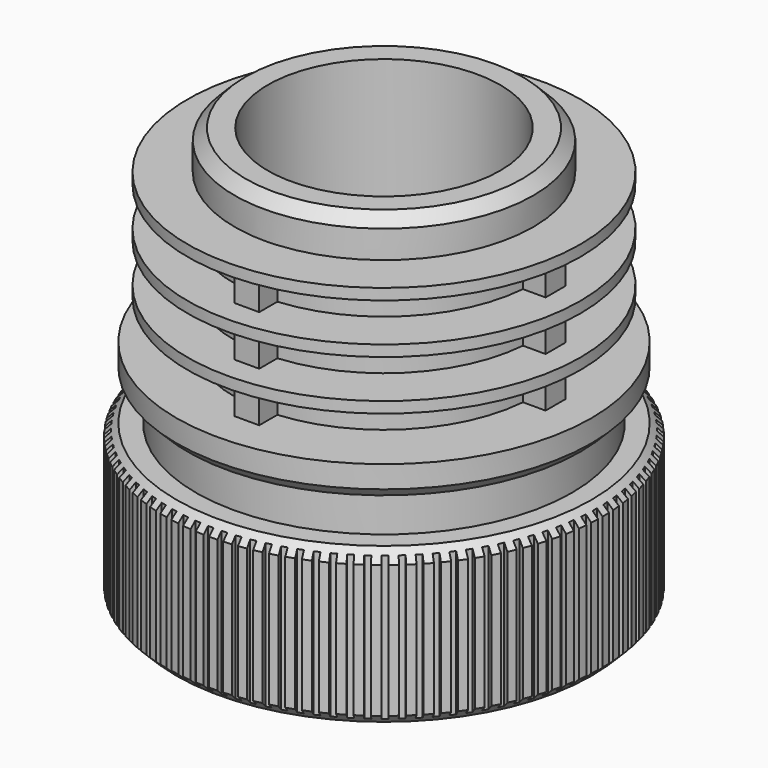
from build123d import *

# Parameters (mm, degrees)
F3_SIZE  = 1
F4_START = -3.5
F4_DEPTH = 21.5
F5_DEPTH = 37.501
F2_R     = 10.5
F6_DEPTH = 33


# Not quite as in the source:
# - a feature names something its author has since deleted; it is built from what else it names


with BuildPart() as f1:
    # F0 (on Front) → F1 (revolve)
    with BuildSketch(Plane.XZ):
        Polygon((0, 0), (19.75, 0), (19.75, 14), (17, 14), (17, 17.5), (18.75, 17.5), (18.75, 20.5), (13.5, 20.5), (13.5, 24), (17.75, 24), (17.75, 25), (13.5, 25), (13.5, 28.5), (17.75, 28.5), (17.75, 29.5), (13.5, 29.5), (13.5, 33), (17.75, 33), (17.75, 34), (13.5, 34), (13.5, 37.5), (0, 37.5), align=None)
    revolve(axis=Axis((0, 0, 18.75), (0, 0, -1)))

    # F3
    f3_edges = [f1.edges().sort_by_distance(p)[0] for p in [
        (-19.75, 0, 14),
        (-18.75, 0, 17.5),
        (-19.75, 0, 0),
        (-13.5, 0, 37.5),
    ]]
    chamfer(f3_edges, length=F3_SIZE)

    # F2 (on face) → F4 (join)
    with BuildSketch(Plane.XY.offset(37.5).offset(F4_START)):
        with BuildLine():
            Line((1.125, -15.5), (1.125, -13.453043336))
            ThreePointArc((1.125, -13.453043336), (0, -13.5), (-1.125, -13.453043336))
            Line((-1.125, -13.453043336), (-1.125, -15.5))
            Line((-1.125, -15.5), (1.125, -15.5))
        make_face()
        with BuildLine():
            ThreePointArc((-13.453043336, -1.125), (-13.5, 0), (-13.453043336, 1.125))
            Line((-13.453043336, 1.125), (-15.5, 1.125))
            Line((-15.5, 1.125), (-15.5, -1.125))
            Line((-15.5, -1.125), (-13.453043336, -1.125))
        make_face()
        with BuildLine():
            ThreePointArc((-1.125, 13.453043336), (0, 13.5), (1.125, 13.453043336))
            Line((1.125, 13.453043336), (1.125, 15.5))
            Line((1.125, 15.5), (-1.125, 15.5))
            Line((-1.125, 15.5), (-1.125, 13.453043336))
        make_face()
        with BuildLine():
            ThreePointArc((13.453043336, 1.125), (13.4882557256, 0.5629897708), (13.5, 0))
            ThreePointArc((13.5, 0), (13.4882557256, -0.5629897708), (13.453043336, -1.125))
            Line((13.453043336, -1.125), (15.5, -1.125))
            Line((15.5, -1.125), (15.5, 1.125))
            Line((15.5, 1.125), (13.453043336, 1.125))
        make_face()
    extrude(amount=-F4_DEPTH)

    # F2 (on face) → F5 (cut, through all)
    with BuildSketch(Plane.XY.offset(37.5)):
        with BuildLine():
            Line((-3.1159466804, 19.0027202338), (-3.2084511899, 19.4876458548))
            ThreePointArc((-3.2084511899, 19.4876458548), (-3.454892922, 19.4454677212), (-3.7007809631, 19.4001732019))
            Line((-3.7007809631, 19.4001732019), (-3.6070903058, 18.9090295765))
            Line((-3.6070903058, 18.9090295765), (-3.1159466804, 19.0027202338))
        make_face()
        with BuildLine():
            ThreePointArc((-16.2668570836, -11.2005294795), (-16.1237633813, -11.4055580497), (-15.9780856389, -11.6087587328))
            Line((-15.9780856389, -11.6087587328), (-15.5735771417, -11.3148661066))
            Line((-15.5735771417, -11.3148661066), (-15.8674697679, -10.9103576094))
            Line((-15.8674697679, -10.9103576094), (-16.2668570836, -11.2005294795))
        make_face()
        with BuildLine():
            ThreePointArc((-13.8799563847, -14.0502423736), (-13.7009787423, -14.2248262381), (-13.5198053421, -14.3971303916))
            Line((-13.5198053421, -14.3971303916), (-13.1775317891, -14.0326460779))
            Line((-13.1775317891, -14.0326460779), (-13.5420161028, -13.6903725249))
            Line((-13.5420161028, -13.6903725249), (-13.8799563847, -14.0502423736))
        make_face()
        with BuildLine():
            ThreePointArc((-12.9703454432, -14.8940471022), (-12.7807587607, -15.0570483661), (-12.5891237975, -15.2176365448))
            Line((-12.5891237975, -15.2176365448), (-12.2704118027, -14.8323799234))
            Line((-12.2704118027, -14.8323799234), (-12.6556684241, -14.5136679286))
            Line((-12.6556684241, -14.5136679286), (-12.9703454432, -14.8940471022))
        make_face()
        with BuildLine():
            ThreePointArc((15.6790718313, -12.0095464739), (15.8298472032, -11.8100989633), (15.9780856389, -11.6087587328))
            Line((15.9780856389, -11.6087587328), (15.5735771417, -11.3148661066))
            Line((15.5735771417, -11.3148661066), (15.2796845156, -11.7193746038))
            Line((15.2796845156, -11.7193746038), (15.6790718313, -12.0095464739))
        make_face()
        with BuildLine():
            ThreePointArc((17.651716969, -8.8588592971), (17.7624489578, -8.6346920629), (17.8703342862, -8.4091410084))
            Line((17.8703342862, -8.4091410084), (17.41792076, -8.1962513626))
            Line((17.41792076, -8.1962513626), (17.2050311142, -8.6486648889))
            Line((17.2050311142, -8.6486648889), (17.651716969, -8.8588592971))
        make_face()
        with BuildLine():
            ThreePointArc((18.1731377154, -7.7330178828), (18.2695756229, -7.5023400723), (18.3630855963, -7.2704599155))
            Line((18.3630855963, -7.2704599155), (17.8981973533, -7.0863976392))
            Line((17.8981973533, -7.0863976392), (17.714135077, -7.5512858821))
            Line((17.714135077, -7.5512858821), (18.1731377154, -7.7330178828))
        make_face()
        with BuildLine():
            Line((0.5, 19.25), (0.5, 19.7436698716))
            ThreePointArc((0.5, 19.7436698716), (0.2500200345, 19.7484174045), (0, 19.75))
            Line((0, 19.75), (0, 19.25))
            Line((0, 19.25), (0.5, 19.25))
        make_face()
        with BuildLine():
            Line((9.7119115665, 16.6280267538), (9.9497388409, 17.06063296))
            ThreePointArc((9.9497388409, 17.06063296), (9.7329668687, 17.1852220217), (9.5146350635, 17.3070569309))
            Line((9.5146350635, 17.3070569309), (9.2737582265, 16.8689035908))
            Line((9.2737582265, 16.8689035908), (9.7119115665, 16.6280267538))
        make_face()
        with BuildLine():
            Line((8.6486648889, 17.2050311142), (8.8588592971, 17.651716969))
            ThreePointArc((8.8588592971, 17.651716969), (8.6346920629, 17.7624489578), (8.4091410084, 17.8703342862))
            Line((8.4091410084, 17.8703342862), (8.1962513626, 17.41792076))
            Line((8.1962513626, 17.41792076), (8.6486648889, 17.2050311142))
        make_face()
        with BuildLine():
            Line((6.4241053999, 18.1533294415), (6.5766577798, 18.6228373898))
            ThreePointArc((6.5766577798, 18.6228373898), (6.340379773, 18.7046006195), (6.1030856389, 18.7833661968))
            Line((6.1030856389, 18.7833661968), (5.9485771417, 18.3078379387))
            Line((5.9485771417, 18.3078379387), (6.4241053999, 18.1533294415))
        make_face()
        with BuildLine():
            Line((5.2715719085, 18.5208809081), (5.3943426132, 18.999041233))
            ThreePointArc((5.3943426132, 18.999041233), (5.1533968913, 19.0658071028), (4.9116252715, 19.1295174323))
            Line((4.9116252715, 19.1295174323), (4.7872803279, 18.6452258517))
            Line((4.7872803279, 18.6452258517), (5.2715719085, 18.5208809081))
        make_face()
        with BuildLine():
            Line((-1.9166073955, 19.1608746171), (-1.9784806368, 19.6506517543))
            ThreePointArc((-1.9784806368, 19.6506517543), (-2.2270844593, 19.6240310541), (-2.4753313629, 19.594265351))
            Line((-2.4753313629, 19.594265351), (-2.4126647461, 19.0982080003))
            Line((-2.4126647461, 19.0982080003), (-1.9166073955, 19.1608746171))
        make_face()
        with BuildLine():
            Line((-4.3029887474, 18.7695707953), (-4.425759452, 19.2477311201))
            ThreePointArc((-4.425759452, 19.2477311201), (-4.6690665007, 19.1901620111), (-4.9116252715, 19.1295174323))
            Line((-4.9116252715, 19.1295174323), (-4.7872803279, 18.6452258517))
            Line((-4.7872803279, 18.6452258517), (-4.3029887474, 18.7695707953))
        make_face()
        with BuildLine():
            ThreePointArc((-15.531471092, -12.1998322005), (-15.3757859019, -12.3954712657), (-15.2176365448, -12.5891237975))
            Line((-15.2176365448, -12.5891237975), (-14.8323799234, -12.2704118027))
            Line((-14.8323799234, -12.2704118027), (-15.1510919183, -11.8851551813))
            Line((-15.1510919183, -11.8851551813), (-15.531471092, -12.1998322005))
        make_face()
        with BuildLine():
            ThreePointArc((-14.7347894795, -13.1509877573), (-14.5671272201, -13.3364652196), (-14.3971303916, -13.5198053421))
            Line((-14.3971303916, -13.5198053421), (-14.0326460779, -13.1775317891))
            Line((-14.0326460779, -13.1775317891), (-14.3749196308, -12.8130474754))
            Line((-14.3749196308, -12.8130474754), (-14.7347894795, -13.1509877573))
        make_face()
        with BuildLine():
            ThreePointArc((12.1998322005, -15.531471092), (12.3954712657, -15.3757859019), (12.5891237975, -15.2176365448))
            Line((12.5891237975, -15.2176365448), (12.2704118027, -14.8323799234))
            Line((12.2704118027, -14.8323799234), (11.8851551813, -15.1510919183))
            Line((11.8851551813, -15.1510919183), (12.1998322005, -15.531471092))
        make_face()
        with BuildLine():
            ThreePointArc((13.1509877573, -14.7347894795), (13.3364652196, -14.5671272201), (13.5198053421, -14.3971303916))
            Line((13.5198053421, -14.3971303916), (13.1775317891, -14.0326460779))
            Line((13.1775317891, -14.0326460779), (12.8130474754, -14.3749196308))
            Line((12.8130474754, -14.3749196308), (13.1509877573, -14.7347894795))
        make_face()
        with BuildLine():
            Line((18.7695707953, 4.3029887474), (19.2477311201, 4.425759452))
            ThreePointArc((19.2477311201, 4.425759452), (19.1901620111, 4.6690665007), (19.1295174323, 4.9116252715))
            Line((19.1295174323, 4.9116252715), (18.6452258517, 4.7872803279))
            Line((18.6452258517, 4.7872803279), (18.7695707953, 4.3029887474))
        make_face()
        with BuildLine():
            ThreePointArc((14.0502423736, -13.8799563847), (14.2248262381, -13.7009787423), (14.3971303916, -13.5198053421))
            Line((14.3971303916, -13.5198053421), (14.0326460779, -13.1775317891))
            Line((14.0326460779, -13.1775317891), (13.6903725249, -13.5420161028))
            Line((13.6903725249, -13.5420161028), (14.0502423736, -13.8799563847))
        make_face()
        with BuildLine():
            ThreePointArc((14.8940471022, -12.9703454432), (15.0570483661, -12.7807587607), (15.2176365448, -12.5891237975))
            Line((15.2176365448, -12.5891237975), (14.8323799234, -12.2704118027))
            Line((14.8323799234, -12.2704118027), (14.5136679286, -12.6556684241))
            Line((14.5136679286, -12.6556684241), (14.8940471022, -12.9703454432))
        make_face()
        with BuildLine():
            Line((-19.25, 0.5), (-19.7436698716, 0.5))
            ThreePointArc((-19.7436698716, 0.5), (-19.7484174045, 0.2500200345), (-19.75, 0))
            Line((-19.75, 0), (-19.25, 0))
            Line((-19.25, 0), (-19.25, 0.5))
        make_face()
        with BuildLine():
            Line((-12.8130474754, 14.3749196308), (-13.1509877573, 14.7347894795))
            ThreePointArc((-13.1509877573, 14.7347894795), (-13.3364652196, 14.5671272201), (-13.5198053421, 14.3971303916))
            Line((-13.5198053421, 14.3971303916), (-13.1775317891, 14.0326460779))
            Line((-13.1775317891, 14.0326460779), (-12.8130474754, 14.3749196308))
        make_face()
        with BuildLine():
            ThreePointArc((-6.5766577798, -18.6228373898), (-6.340379773, -18.7046006195), (-6.1030856389, -18.7833661968))
            Line((-6.1030856389, -18.7833661968), (-5.9485771417, -18.3078379387))
            Line((-5.9485771417, -18.3078379387), (-6.4241053999, -18.1533294415))
            Line((-6.4241053999, -18.1533294415), (-6.5766577798, -18.6228373898))
        make_face()
        with BuildLine():
            Line((-0.7097041367, 19.243409782), (-0.7407019244, 19.7361055089))
            ThreePointArc((-0.7407019244, 19.7361055089), (-0.9904867117, 19.7251473017), (-1.2401127607, 19.7110278865))
            Line((-1.2401127607, 19.7110278865), (-1.2087175009, 19.2120145222))
            Line((-1.2087175009, 19.2120145222), (-0.7097041367, 19.243409782))
        make_face()
        with BuildLine():
            Line((7.5512858821, 17.714135077), (7.7330178828, 18.1731377154))
            ThreePointArc((7.7330178828, 18.1731377154), (7.5023400723, 18.2695756229), (7.2704599155, 18.3630855963))
            Line((7.2704599155, 18.3630855963), (7.0863976392, 17.8981973533))
            Line((7.0863976392, 17.8981973533), (7.5512858821, 17.714135077))
        make_face()
        with BuildLine():
            ThreePointArc((-1.7387286529, -19.6733149894), (-1.4895400657, -19.693749526), (-1.2401127607, -19.7110278865))
            Line((-1.2401127607, -19.7110278865), (-1.2087175009, -19.2120145222))
            Line((-1.2087175009, -19.2120145222), (-1.7077308652, -19.1806192625))
            Line((-1.7077308652, -19.1806192625), (-1.7387286529, -19.6733149894))
        make_face()
        with BuildLine():
            ThreePointArc((-4.1907384407, -19.3002645402), (-3.9460759065, -19.3517695558), (-3.7007809631, -19.4001732019))
            Line((-3.7007809631, -19.4001732019), (-3.6070903058, -18.9090295765))
            Line((-3.6070903058, -18.9090295765), (-4.0982339311, -18.8153389192))
            Line((-4.0982339311, -18.8153389192), (-4.1907384407, -19.3002645402))
        make_face()
        with BuildLine():
            ThreePointArc((18.999041233, -5.3943426132), (19.0658071028, -5.1533968913), (19.1295174323, -4.9116252715))
            Line((19.1295174323, -4.9116252715), (18.6452258517, -4.7872803279))
            Line((18.6452258517, -4.7872803279), (18.5208809081, -5.2715719085))
            Line((18.5208809081, -5.2715719085), (18.999041233, -5.3943426132))
        make_face()
        with BuildLine():
            ThreePointArc((-16.938045222, -10.1570233857), (-16.8081077328, -10.3706323067), (-16.6754765287, -10.5825792008))
            Line((-16.6754765287, -10.5825792008), (-16.2533125659, -10.3146658033))
            Line((-16.2533125659, -10.3146658033), (-16.5212259634, -9.8925018406))
            Line((-16.5212259634, -9.8925018406), (-16.938045222, -10.1570233857))
        make_face()
        with BuildLine():
            ThreePointArc((19.6733149894, -1.7387286529), (19.693749526, -1.4895400657), (19.7110278865, -1.2401127607))
            Line((19.7110278865, -1.2401127607), (19.2120145222, -1.2087175009))
            Line((19.2120145222, -1.2087175009), (19.1806192625, -1.7077308652))
            Line((19.1806192625, -1.7077308652), (19.6733149894, -1.7387286529))
        make_face()
        with BuildLine():
            ThreePointArc((10.1570233857, -16.938045222), (10.3706323067, -16.8081077328), (10.5825792008, -16.6754765287))
            Line((10.5825792008, -16.6754765287), (10.3146658033, -16.2533125659))
            Line((10.3146658033, -16.2533125659), (9.8925018406, -16.5212259634))
            Line((9.8925018406, -16.5212259634), (10.1570233857, -16.938045222))
        make_face()
        with BuildLine():
            Line((19.243409782, 0.7097041367), (19.7361055089, 0.7407019244))
            ThreePointArc((19.7361055089, 0.7407019244), (19.7251473017, 0.9904867117), (19.7110278865, 1.2401127607))
            Line((19.7110278865, 1.2401127607), (19.2120145222, 1.2087175009))
            Line((19.2120145222, 1.2087175009), (19.243409782, 0.7097041367))
        make_face()
        with BuildLine():
            Line((-5.4730488836, 18.4623464359), (-5.6256012635, 18.9318543842))
            ThreePointArc((-5.6256012635, 18.9318543842), (-5.864813407, 18.8591214986), (-6.1030856389, 18.7833661968))
            Line((-6.1030856389, 18.7833661968), (-5.9485771417, 18.3078379387))
            Line((-5.9485771417, 18.3078379387), (-5.4730488836, 18.4623464359))
        make_face()
        with BuildLine():
            Line((-7.7438378364, 17.6308104058), (-7.9540322446, 18.0774962606))
            ThreePointArc((-7.9540322446, 18.0774962606), (-8.1822422812, 17.9753556641), (-8.4091410084, 17.8703342862))
            Line((-8.4091410084, 17.8703342862), (-8.1962513626, 17.41792076))
            Line((-8.1962513626, 17.41792076), (-7.7438378364, 17.6308104058))
        make_face()
        with BuildLine():
            ThreePointArc((-12.0095464739, -15.6790718313), (-11.8100989633, -15.8298472032), (-11.6087587328, -15.9780856389))
            Line((-11.6087587328, -15.9780856389), (-11.3148661066, -15.5735771417))
            Line((-11.3148661066, -15.5735771417), (-11.7193746038, -15.2796845156))
            Line((-11.7193746038, -15.2796845156), (-12.0095464739, -15.6790718313))
        make_face()
        with BuildLine():
            Line((18.4623464359, 5.4730488836), (18.9318543842, 5.6256012635))
            ThreePointArc((18.9318543842, 5.6256012635), (18.8591214986, 5.864813407), (18.7833661968, 6.1030856389))
            Line((18.7833661968, 6.1030856389), (18.3078379387, 5.9485771417))
            Line((18.3078379387, 5.9485771417), (18.4623464359, 5.4730488836))
        make_face()
        with BuildLine():
            Line((-9.8925018406, 16.5212259634), (-10.1570233857, 16.938045222))
            ThreePointArc((-10.1570233857, 16.938045222), (-10.3706323067, 16.8081077328), (-10.5825792008, 16.6754765287))
            Line((-10.5825792008, 16.6754765287), (-10.3146658033, 16.2533125659))
            Line((-10.3146658033, 16.2533125659), (-9.8925018406, 16.5212259634))
        make_face()
        with BuildLine():
            ThreePointArc((17.06063296, -9.9497388409), (17.1852220217, -9.7329668687), (17.3070569309, -9.5146350635))
            Line((17.3070569309, -9.5146350635), (16.8689035908, -9.2737582265))
            Line((16.8689035908, -9.2737582265), (16.6280267538, -9.7119115665))
            Line((16.6280267538, -9.7119115665), (17.06063296, -9.9497388409))
        make_face()
        with BuildLine():
            ThreePointArc((-19.4876458548, -3.2084511899), (-19.4454677212, -3.454892922), (-19.4001732019, -3.7007809631))
            Line((-19.4001732019, -3.7007809631), (-18.9090295765, -3.6070903058))
            Line((-18.9090295765, -3.6070903058), (-19.0027202338, -3.1159466804))
            Line((-19.0027202338, -3.1159466804), (-19.4876458548, -3.2084511899))
        make_face()
        with BuildLine():
            ThreePointArc((-19.2477311201, -4.425759452), (-19.1901620111, -4.6690665007), (-19.1295174323, -4.9116252715))
            Line((-19.1295174323, -4.9116252715), (-18.6452258517, -4.7872803279))
            Line((-18.6452258517, -4.7872803279), (-18.7695707953, -4.3029887474))
            Line((-18.7695707953, -4.3029887474), (-19.2477311201, -4.425759452))
        make_face()
        with BuildLine():
            Line((-13.6903725249, 13.5420161028), (-14.0502423736, 13.8799563847))
            ThreePointArc((-14.0502423736, 13.8799563847), (-14.2248262381, 13.7009787423), (-14.3971303916, 13.5198053421))
            Line((-14.3971303916, 13.5198053421), (-14.0326460779, 13.1775317891))
            Line((-14.0326460779, 13.1775317891), (-13.6903725249, 13.5420161028))
        make_face()
        with BuildLine():
            ThreePointArc((3.2084511899, -19.4876458548), (3.454892922, -19.4454677212), (3.7007809631, -19.4001732019))
            Line((3.7007809631, -19.4001732019), (3.6070903058, -18.9090295765))
            Line((3.6070903058, -18.9090295765), (3.1159466804, -19.0027202338))
            Line((3.1159466804, -19.0027202338), (3.2084511899, -19.4876458548))
        make_face()
        with BuildLine():
            ThreePointArc((-5.3943426132, -18.999041233), (-5.1533968913, -19.0658071028), (-4.9116252715, -19.1295174323))
            Line((-4.9116252715, -19.1295174323), (-4.7872803279, -18.6452258517))
            Line((-4.7872803279, -18.6452258517), (-5.2715719085, -18.5208809081))
            Line((-5.2715719085, -18.5208809081), (-5.3943426132, -18.999041233))
        make_face()
        with BuildLine():
            Line((1.7077308652, 19.1806192625), (1.7387286529, 19.6733149894))
            ThreePointArc((1.7387286529, 19.6733149894), (1.4895400657, 19.693749526), (1.2401127607, 19.7110278865))
            Line((1.2401127607, 19.7110278865), (1.2087175009, 19.2120145222))
            Line((1.2087175009, 19.2120145222), (1.7077308652, 19.1806192625))
        make_face()
        with BuildLine():
            Line((13.5420161028, 13.6903725249), (13.8799563847, 14.0502423736))
            ThreePointArc((13.8799563847, 14.0502423736), (13.7009787423, 14.2248262381), (13.5198053421, 14.3971303916))
            Line((13.5198053421, 14.3971303916), (13.1775317891, 14.0326460779))
            Line((13.1775317891, 14.0326460779), (13.5420161028, 13.6903725249))
        make_face()
        with BuildLine():
            ThreePointArc((19.5253185208, -2.9705953381), (19.5613594153, -2.7231815629), (19.594265351, -2.4753313629))
            Line((19.594265351, -2.4753313629), (19.0982080003, -2.4126647461))
            Line((19.0982080003, -2.4126647461), (19.0355413835, -2.9087220968))
            Line((19.0355413835, -2.9087220968), (19.5253185208, -2.9705953381))
        make_face()
        with BuildLine():
            ThreePointArc((5.6256012635, -18.9318543842), (5.864813407, -18.8591214986), (6.1030856389, -18.7833661968))
            Line((6.1030856389, -18.7833661968), (5.9485771417, -18.3078379387))
            Line((5.9485771417, -18.3078379387), (5.4730488836, -18.4623464359))
            Line((5.4730488836, -18.4623464359), (5.6256012635, -18.9318543842))
        make_face()
        with BuildLine():
            ThreePointArc((-2.9705953381, -19.5253185208), (-2.7231815629, -19.5613594153), (-2.4753313629, -19.594265351))
            Line((-2.4753313629, -19.594265351), (-2.4126647461, -19.0982080003))
            Line((-2.4126647461, -19.0982080003), (-2.9087220968, -19.0355413835))
            Line((-2.9087220968, -19.0355413835), (-2.9705953381, -19.5253185208))
        make_face()
        with BuildLine():
            Line((-6.6215093962, 18.0822596297), (-6.8032413969, 18.5412622681))
            ThreePointArc((-6.8032413969, 18.5412622681), (-7.0374145742, 18.4536526496), (-7.2704599155, 18.3630855963))
            Line((-7.2704599155, 18.3630855963), (-7.0863976392, 17.8981973533))
            Line((-7.0863976392, 17.8981973533), (-6.6215093962, 18.0822596297))
        make_face()
        with BuildLine():
            Line((19.0027202338, 3.1159466804), (19.4876458548, 3.2084511899))
            ThreePointArc((19.4876458548, 3.2084511899), (19.4454677212, 3.454892922), (19.4001732019, 3.7007809631))
            Line((19.4001732019, 3.7007809631), (18.9090295765, 3.6070903058))
            Line((18.9090295765, 3.6070903058), (19.0027202338, 3.1159466804))
        make_face()
        with BuildLine():
            Line((-8.8356048864, 17.1097804279), (-9.0734321609, 17.5423866341))
            ThreePointArc((-9.0734321609, 17.5423866341), (-9.294778416, 17.4261181621), (-9.5146350635, 17.3070569309))
            Line((-9.5146350635, 17.3070569309), (-9.2737582265, 16.8689035908))
            Line((-9.2737582265, 16.8689035908), (-8.8356048864, 17.1097804279))
        make_face()
        with BuildLine():
            ThreePointArc((-19.7361055089, -0.7407019244), (-19.7251473017, -0.9904867117), (-19.7110278865, -1.2401127607))
            Line((-19.7110278865, -1.2401127607), (-19.2120145222, -1.2087175009))
            Line((-19.2120145222, -1.2087175009), (-19.243409782, -0.7097041367))
            Line((-19.243409782, -0.7097041367), (-19.7361055089, -0.7407019244))
        make_face()
        with BuildLine():
            Line((-10.9103576094, 15.8674697679), (-11.2005294795, 16.2668570836))
            ThreePointArc((-11.2005294795, 16.2668570836), (-11.4055580497, 16.1237633813), (-11.6087587328, 15.9780856389))
            Line((-11.6087587328, 15.9780856389), (-11.3148661066, 15.5735771417))
            Line((-11.3148661066, 15.5735771417), (-10.9103576094, 15.8674697679))
        make_face()
        with BuildLine():
            ThreePointArc((-18.9318543842, -5.6256012635), (-18.8591214986, -5.864813407), (-18.7833661968, -6.1030856389))
            Line((-18.7833661968, -6.1030856389), (-18.3078379387, -5.9485771417))
            Line((-18.3078379387, -5.9485771417), (-18.4623464359, -5.4730488836))
            Line((-18.4623464359, -5.4730488836), (-18.9318543842, -5.6256012635))
        make_face()
        with BuildLine():
            Line((11.7193746038, 15.2796845156), (12.0095464739, 15.6790718313))
            ThreePointArc((12.0095464739, 15.6790718313), (11.8100989633, 15.8298472032), (11.6087587328, 15.9780856389))
            Line((11.6087587328, 15.9780856389), (11.3148661066, 15.5735771417))
            Line((11.3148661066, 15.5735771417), (11.7193746038, 15.2796845156))
        make_face()
        with BuildLine():
            Line((4.0982339311, 18.8153389192), (4.1907384407, 19.3002645402))
            ThreePointArc((4.1907384407, 19.3002645402), (3.9460759065, 19.3517695558), (3.7007809631, 19.4001732019))
            Line((3.7007809631, 19.4001732019), (3.6070903058, 18.9090295765))
            Line((3.6070903058, 18.9090295765), (4.0982339311, 18.8153389192))
        make_face()
        with BuildLine():
            ThreePointArc((9.0734321609, -17.5423866341), (9.294778416, -17.4261181621), (9.5146350635, -17.3070569309))
            Line((9.5146350635, -17.3070569309), (9.2737582265, -16.8689035908))
            Line((9.2737582265, -16.8689035908), (8.8356048864, -17.1097804279))
            Line((8.8356048864, -17.1097804279), (9.0734321609, -17.5423866341))
        make_face()
        with BuildLine():
            ThreePointArc((19.7436698716, -0.5), (19.7484174045, -0.2500200345), (19.75, 0))
            Line((19.75, 0), (19.25, 0))
            Line((19.25, 0), (19.25, -0.5))
            Line((19.25, -0.5), (19.7436698716, -0.5))
        make_face()
        with BuildLine():
            Line((19.1608746171, 1.9166073955), (19.6506517543, 1.9784806368))
            ThreePointArc((19.6506517543, 1.9784806368), (19.6240310541, 2.2270844593), (19.594265351, 2.4753313629))
            Line((19.594265351, 2.4753313629), (19.0982080003, 2.4126647461))
            Line((19.0982080003, 2.4126647461), (19.1608746171, 1.9166073955))
        make_face()
        with BuildLine():
            Line((15.8674697679, 10.9103576094), (16.2668570836, 11.2005294795))
            ThreePointArc((16.2668570836, 11.2005294795), (16.1237633813, 11.4055580497), (15.9780856389, 11.6087587328))
            Line((15.9780856389, 11.6087587328), (15.5735771417, 11.3148661066))
            Line((15.5735771417, 11.3148661066), (15.8674697679, 10.9103576094))
        make_face()
        with BuildLine():
            Line((14.3749196308, 12.8130474754), (14.7347894795, 13.1509877573))
            ThreePointArc((14.7347894795, 13.1509877573), (14.5671272201, 13.3364652196), (14.3971303916, 13.5198053421))
            Line((14.3971303916, 13.5198053421), (14.0326460779, 13.1775317891))
            Line((14.0326460779, 13.1775317891), (14.3749196308, 12.8130474754))
        make_face()
        with BuildLine():
            Line((12.6556684241, 14.5136679286), (12.9703454432, 14.8940471022))
            ThreePointArc((12.9703454432, 14.8940471022), (12.7807587607, 15.0570483661), (12.5891237975, 15.2176365448))
            Line((12.5891237975, 15.2176365448), (12.2704118027, 14.8323799234))
            Line((12.2704118027, 14.8323799234), (12.6556684241, 14.5136679286))
        make_face()
        with BuildLine():
            Line((10.7368297661, 15.9853991684), (11.0013513112, 16.402218427))
            ThreePointArc((11.0013513112, 16.402218427), (10.7928301008, 16.5401728653), (10.5825792008, 16.6754765287))
            Line((10.5825792008, 16.6754765287), (10.3146658033, 16.2533125659))
            Line((10.3146658033, 16.2533125659), (10.7368297661, 15.9853991684))
        make_face()
        with BuildLine():
            Line((18.0822596297, 6.6215093962), (18.5412622681, 6.8032413969))
            ThreePointArc((18.5412622681, 6.8032413969), (18.4536526496, 7.0374145742), (18.3630855963, 7.2704599155))
            Line((18.3630855963, 7.2704599155), (17.8981973533, 7.0863976392))
            Line((17.8981973533, 7.0863976392), (18.0822596297, 6.6215093962))
        make_face()
        with BuildLine():
            Line((17.1097804279, 8.8356048864), (17.5423866341, 9.0734321609))
            ThreePointArc((17.5423866341, 9.0734321609), (17.4261181621, 9.294778416), (17.3070569309, 9.5146350635))
            Line((17.3070569309, 9.5146350635), (16.8689035908, 9.2737582265))
            Line((16.8689035908, 9.2737582265), (17.1097804279, 8.8356048864))
        make_face()
        with BuildLine():
            ThreePointArc((-7.7330178828, -18.1731377154), (-7.5023400723, -18.2695756229), (-7.2704599155, -18.3630855963))
            Line((-7.2704599155, -18.3630855963), (-7.0863976392, -17.8981973533))
            Line((-7.0863976392, -17.8981973533), (-7.5512858821, -17.714135077))
            Line((-7.5512858821, -17.714135077), (-7.7330178828, -18.1731377154))
        make_face()
        with BuildLine():
            Line((16.5212259634, 9.8925018406), (16.938045222, 10.1570233857))
            ThreePointArc((16.938045222, 10.1570233857), (16.8081077328, 10.3706323067), (16.6754765287, 10.5825792008))
            Line((16.6754765287, 10.5825792008), (16.2533125659, 10.3146658033))
            Line((16.2533125659, 10.3146658033), (16.5212259634, 9.8925018406))
        make_face()
        with BuildLine():
            Line((15.1510919183, 11.8851551813), (15.531471092, 12.1998322005))
            ThreePointArc((15.531471092, 12.1998322005), (15.3757859019, 12.3954712657), (15.2176365448, 12.5891237975))
            Line((15.2176365448, 12.5891237975), (14.8323799234, 12.2704118027))
            Line((14.8323799234, 12.2704118027), (15.1510919183, 11.8851551813))
        make_face()
        with BuildLine():
            ThreePointArc((-0.5, -19.7436698716), (-0.2500200345, -19.7484174045), (0, -19.75))
            Line((0, -19.75), (0, -19.25))
            Line((0, -19.25), (-0.5, -19.25))
            Line((-0.5, -19.25), (-0.5, -19.7436698716))
        make_face()
        with BuildLine():
            Line((-15.2796845156, 11.7193746038), (-15.6790718313, 12.0095464739))
            ThreePointArc((-15.6790718313, 12.0095464739), (-15.8298472032, 11.8100989633), (-15.9780856389, 11.6087587328))
            Line((-15.9780856389, 11.6087587328), (-15.5735771417, 11.3148661066))
            Line((-15.5735771417, 11.3148661066), (-15.2796845156, 11.7193746038))
        make_face()
        with BuildLine():
            Line((-18.8153389192, 4.0982339311), (-19.3002645402, 4.1907384407))
            ThreePointArc((-19.3002645402, 4.1907384407), (-19.3517695558, 3.9460759065), (-19.4001732019, 3.7007809631))
            Line((-19.4001732019, 3.7007809631), (-18.9090295765, 3.6070903058))
            Line((-18.9090295765, 3.6070903058), (-18.8153389192, 4.0982339311))
        make_face()
        with BuildLine():
            Line((-19.1806192625, 1.7077308652), (-19.6733149894, 1.7387286529))
            ThreePointArc((-19.6733149894, 1.7387286529), (-19.693749526, 1.4895400657), (-19.7110278865, 1.2401127607))
            Line((-19.7110278865, 1.2401127607), (-19.2120145222, 1.2087175009))
            Line((-19.2120145222, 1.2087175009), (-19.1806192625, 1.7077308652))
        make_face()
        with BuildLine():
            ThreePointArc((0.7407019244, -19.7361055089), (0.9904867117, -19.7251473017), (1.2401127607, -19.7110278865))
            Line((1.2401127607, -19.7110278865), (1.2087175009, -19.2120145222))
            Line((1.2087175009, -19.2120145222), (0.7097041367, -19.243409782))
            Line((0.7097041367, -19.243409782), (0.7407019244, -19.7361055089))
        make_face()
        with BuildLine():
            Line((-15.9853991684, 10.7368297661), (-16.402218427, 11.0013513112))
            ThreePointArc((-16.402218427, 11.0013513112), (-16.5401728653, 10.7928301008), (-16.6754765287, 10.5825792008))
            Line((-16.6754765287, 10.5825792008), (-16.2533125659, 10.3146658033))
            Line((-16.2533125659, 10.3146658033), (-15.9853991684, 10.7368297661))
        make_face()
        with BuildLine():
            Line((-18.1533294415, 6.4241053999), (-18.6228373898, 6.5766577798))
            ThreePointArc((-18.6228373898, 6.5766577798), (-18.7046006195, 6.340379773), (-18.7833661968, 6.1030856389))
            Line((-18.7833661968, 6.1030856389), (-18.3078379387, 5.9485771417))
            Line((-18.3078379387, 5.9485771417), (-18.1533294415, 6.4241053999))
        make_face()
        with BuildLine():
            ThreePointArc((1.9784806368, -19.6506517543), (2.2270844593, -19.6240310541), (2.4753313629, -19.594265351))
            Line((2.4753313629, -19.594265351), (2.4126647461, -19.0982080003))
            Line((2.4126647461, -19.0982080003), (1.9166073955, -19.1608746171))
            Line((1.9166073955, -19.1608746171), (1.9784806368, -19.6506517543))
        make_face()
        with BuildLine():
            Line((-16.6280267538, 9.7119115665), (-17.06063296, 9.9497388409))
            ThreePointArc((-17.06063296, 9.9497388409), (-17.1852220217, 9.7329668687), (-17.3070569309, 9.5146350635))
            Line((-17.3070569309, 9.5146350635), (-16.8689035908, 9.2737582265))
            Line((-16.8689035908, 9.2737582265), (-16.6280267538, 9.7119115665))
        make_face()
        with BuildLine():
            Line((-17.714135077, 7.5512858821), (-18.1731377154, 7.7330178828))
            ThreePointArc((-18.1731377154, 7.7330178828), (-18.2695756229, 7.5023400723), (-18.3630855963, 7.2704599155))
            Line((-18.3630855963, 7.2704599155), (-17.8981973533, 7.0863976392))
            Line((-17.8981973533, 7.0863976392), (-17.714135077, 7.5512858821))
        make_face()
        with BuildLine():
            Line((-18.5208809081, 5.2715719085), (-18.999041233, 5.3943426132))
            ThreePointArc((-18.999041233, 5.3943426132), (-19.0658071028, 5.1533968913), (-19.1295174323, 4.9116252715))
            Line((-19.1295174323, 4.9116252715), (-18.6452258517, 4.7872803279))
            Line((-18.6452258517, 4.7872803279), (-18.5208809081, 5.2715719085))
        make_face()
        with BuildLine():
            Line((-17.2050311142, 8.6486648889), (-17.651716969, 8.8588592971))
            ThreePointArc((-17.651716969, 8.8588592971), (-17.7624489578, 8.6346920629), (-17.8703342862, 8.4091410084))
            Line((-17.8703342862, 8.4091410084), (-17.41792076, 8.1962513626))
            Line((-17.41792076, 8.1962513626), (-17.2050311142, 8.6486648889))
        make_face()
        with BuildLine():
            Line((2.9087220968, 19.0355413835), (2.9705953381, 19.5253185208))
            ThreePointArc((2.9705953381, 19.5253185208), (2.7231815629, 19.5613594153), (2.4753313629, 19.594265351))
            Line((2.4753313629, 19.594265351), (2.4126647461, 19.0982080003))
            Line((2.4126647461, 19.0982080003), (2.9087220968, 19.0355413835))
        make_face()
        with BuildLine():
            Line((17.6308104058, 7.7438378364), (18.0774962606, 7.9540322446))
            ThreePointArc((18.0774962606, 7.9540322446), (17.9753556641, 8.1822422812), (17.8703342862, 8.4091410084))
            Line((17.8703342862, 8.4091410084), (17.41792076, 8.1962513626))
            Line((17.41792076, 8.1962513626), (17.6308104058, 7.7438378364))
        make_face()
        with BuildLine():
            ThreePointArc((19.3002645402, -4.1907384407), (19.3517695558, -3.9460759065), (19.4001732019, -3.7007809631))
            Line((19.4001732019, -3.7007809631), (18.9090295765, -3.6070903058))
            Line((18.9090295765, -3.6070903058), (18.8153389192, -4.0982339311))
            Line((18.8153389192, -4.0982339311), (19.3002645402, -4.1907384407))
        make_face()
        with BuildLine():
            ThreePointArc((18.6228373898, -6.5766577798), (18.7046006195, -6.340379773), (18.7833661968, -6.1030856389))
            Line((18.7833661968, -6.1030856389), (18.3078379387, -5.9485771417))
            Line((18.3078379387, -5.9485771417), (18.1533294415, -6.4241053999))
            Line((18.1533294415, -6.4241053999), (18.6228373898, -6.5766577798))
        make_face()
        with BuildLine():
            ThreePointArc((16.402218427, -11.0013513112), (16.5401728653, -10.7928301008), (16.6754765287, -10.5825792008))
            Line((16.6754765287, -10.5825792008), (16.2533125659, -10.3146658033))
            Line((16.2533125659, -10.3146658033), (15.9853991684, -10.7368297661))
            Line((15.9853991684, -10.7368297661), (16.402218427, -11.0013513112))
        make_face()
        with BuildLine():
            ThreePointArc((11.2005294795, -16.2668570836), (11.4055580497, -16.1237633813), (11.6087587328, -15.9780856389))
            Line((11.6087587328, -15.9780856389), (11.3148661066, -15.5735771417))
            Line((11.3148661066, -15.5735771417), (10.9103576094, -15.8674697679))
            Line((10.9103576094, -15.8674697679), (11.2005294795, -16.2668570836))
        make_face()
        with BuildLine():
            ThreePointArc((7.9540322446, -18.0774962606), (8.1822422812, -17.9753556641), (8.4091410084, -17.8703342862))
            Line((8.4091410084, -17.8703342862), (8.1962513626, -17.41792076))
            Line((8.1962513626, -17.41792076), (7.7438378364, -17.6308104058))
            Line((7.7438378364, -17.6308104058), (7.9540322446, -18.0774962606))
        make_face()
        with BuildLine():
            ThreePointArc((6.8032413969, -18.5412622681), (7.0374145742, -18.4536526496), (7.2704599155, -18.3630855963))
            Line((7.2704599155, -18.3630855963), (7.0863976392, -17.8981973533))
            Line((7.0863976392, -17.8981973533), (6.6215093962, -18.0822596297))
            Line((6.6215093962, -18.0822596297), (6.8032413969, -18.5412622681))
        make_face()
        with BuildLine():
            ThreePointArc((4.425759452, -19.2477311201), (4.6690665007, -19.1901620111), (4.9116252715, -19.1295174323))
            Line((4.9116252715, -19.1295174323), (4.7872803279, -18.6452258517))
            Line((4.7872803279, -18.6452258517), (4.3029887474, -18.7695707953))
            Line((4.3029887474, -18.7695707953), (4.425759452, -19.2477311201))
        make_face()
        with BuildLine():
            ThreePointArc((-8.8588592971, -17.651716969), (-8.6346920629, -17.7624489578), (-8.4091410084, -17.8703342862))
            Line((-8.4091410084, -17.8703342862), (-8.1962513626, -17.41792076))
            Line((-8.1962513626, -17.41792076), (-8.6486648889, -17.2050311142))
            Line((-8.6486648889, -17.2050311142), (-8.8588592971, -17.651716969))
        make_face()
        with BuildLine():
            ThreePointArc((-9.9497388409, -17.06063296), (-9.7329668687, -17.1852220217), (-9.5146350635, -17.3070569309))
            Line((-9.5146350635, -17.3070569309), (-9.2737582265, -16.8689035908))
            Line((-9.2737582265, -16.8689035908), (-9.7119115665, -16.6280267538))
            Line((-9.7119115665, -16.6280267538), (-9.9497388409, -17.06063296))
        make_face()
        with BuildLine():
            ThreePointArc((-11.0013513112, -16.402218427), (-10.7928301008, -16.5401728653), (-10.5825792008, -16.6754765287))
            Line((-10.5825792008, -16.6754765287), (-10.3146658033, -16.2533125659))
            Line((-10.3146658033, -16.2533125659), (-10.7368297661, -15.9853991684))
            Line((-10.7368297661, -15.9853991684), (-11.0013513112, -16.402218427))
        make_face()
        with BuildLine():
            ThreePointArc((-17.5423866341, -9.0734321609), (-17.4261181621, -9.294778416), (-17.3070569309, -9.5146350635))
            Line((-17.3070569309, -9.5146350635), (-16.8689035908, -9.2737582265))
            Line((-16.8689035908, -9.2737582265), (-17.1097804279, -8.8356048864))
            Line((-17.1097804279, -8.8356048864), (-17.5423866341, -9.0734321609))
        make_face()
        with BuildLine():
            ThreePointArc((-18.0774962606, -7.9540322446), (-17.9753556641, -8.1822422812), (-17.8703342862, -8.4091410084))
            Line((-17.8703342862, -8.4091410084), (-17.41792076, -8.1962513626))
            Line((-17.41792076, -8.1962513626), (-17.6308104058, -7.7438378364))
            Line((-17.6308104058, -7.7438378364), (-18.0774962606, -7.9540322446))
        make_face()
        with BuildLine():
            ThreePointArc((-18.5412622681, -6.8032413969), (-18.4536526496, -7.0374145742), (-18.3630855963, -7.2704599155))
            Line((-18.3630855963, -7.2704599155), (-17.8981973533, -7.0863976392))
            Line((-17.8981973533, -7.0863976392), (-18.0822596297, -6.6215093962))
            Line((-18.0822596297, -6.6215093962), (-18.5412622681, -6.8032413969))
        make_face()
        with BuildLine():
            ThreePointArc((-19.6506517543, -1.9784806368), (-19.6240310541, -2.2270844593), (-19.594265351, -2.4753313629))
            Line((-19.594265351, -2.4753313629), (-19.0982080003, -2.4126647461))
            Line((-19.0982080003, -2.4126647461), (-19.1608746171, -1.9166073955))
            Line((-19.1608746171, -1.9166073955), (-19.6506517543, -1.9784806368))
        make_face()
        with BuildLine():
            Line((-19.0355413835, 2.9087220968), (-19.5253185208, 2.9705953381))
            ThreePointArc((-19.5253185208, 2.9705953381), (-19.5613594153, 2.7231815629), (-19.594265351, 2.4753313629))
            Line((-19.594265351, 2.4753313629), (-19.0982080003, 2.4126647461))
            Line((-19.0982080003, 2.4126647461), (-19.0355413835, 2.9087220968))
        make_face()
        with BuildLine():
            Line((-11.8851551813, 15.1510919183), (-12.1998322005, 15.531471092))
            ThreePointArc((-12.1998322005, 15.531471092), (-12.3954712657, 15.3757859019), (-12.5891237975, 15.2176365448))
            Line((-12.5891237975, 15.2176365448), (-12.2704118027, 14.8323799234))
            Line((-12.2704118027, 14.8323799234), (-11.8851551813, 15.1510919183))
        make_face()
        with BuildLine():
            Line((-14.5136679286, 12.6556684241), (-14.8940471022, 12.9703454432))
            ThreePointArc((-14.8940471022, 12.9703454432), (-15.0570483661, 12.7807587607), (-15.2176365448, 12.5891237975))
            Line((-15.2176365448, 12.5891237975), (-14.8323799234, 12.2704118027))
            Line((-14.8323799234, 12.2704118027), (-14.5136679286, 12.6556684241))
        make_face()
    extrude(amount=-F5_DEPTH, mode=Mode.SUBTRACT)

    # F2 (on face) → F6 (cut)
    with BuildSketch(Plane.XY.offset(37.5)):
        Circle(F2_R)
    extrude(amount=-F6_DEPTH, mode=Mode.SUBTRACT)


solid = f1.part
